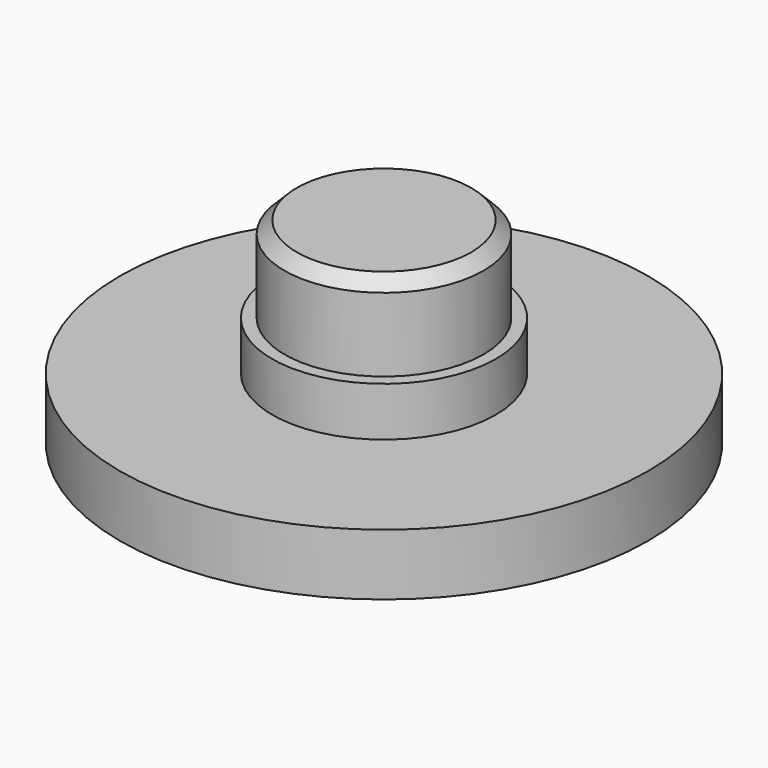
from build123d import *

# Parameters (mm, degrees)
F0_R     = 10.75
F0_R_2   = 10
F1_DEPTH = 2.5
F2_R     = 4.05
F3_DEPTH = 5.5
F4_SIZE  = 0.5
F5_R     = 4.55
F6_DEPTH = 2
F7_DEPTH = 0.5


# Not quite as in the source:
# - a feature names something its author has since deleted; it is built from what else it names


with BuildPart() as f1:
    # F0 (on Top) → F1 (new body)
    with BuildSketch(Plane.XY):
        Circle(F0_R)
        Circle(F0_R_2, mode=Mode.SUBTRACT)
        Circle(F0_R_2)
        Polygon((-0.8144098687, 5.5770273648), (3.432810713, 8.7260752933), (2.0940857055, 4.3571935282), (5.0940976108, -0.8390625077), (5.23705231, -2.0832140472), (5.8405975225, -7.3359389308), (2.7263974316, -3.992128183), (-3.2736025686, -3.992128183), (-4.4226424415, -3.4938133181), (-9.2734082358, -1.3901363628), (-4.8204831373, -0.3650653455), (-1.8204831373, 4.8310870772), align=None, mode=Mode.SUBTRACT)
        Polygon((2.0940857055, 4.3571935282), (3.432810713, 8.7260752933), (-0.8144098687, 5.5770273648), (-1.8204831373, 4.8310870772), (-4.8204831373, -0.3650653455), (-9.2734082358, -1.3901363628), (-4.4226424415, -3.4938133181), (-3.2736025686, -3.992128183), (2.7263974316, -3.992128183), (5.8405975225, -7.3359389308), (5.23705231, -2.0832140472), (5.0940976108, -0.8390625077), align=None)
    extrude(amount=F1_DEPTH)

    # F2 (on face) → F3 (join)
    with BuildSketch(Plane.XY.offset(2.5)):
        Circle(F2_R)
    extrude(amount=F3_DEPTH)

    # F4
    f4_edges = [f1.edges().sort_by_distance(p)[0] for p in [
        (-4.05, 0, 8),
    ]]
    chamfer(f4_edges, length=F4_SIZE)

    # F5 (on face) → F6 (join)
    with BuildSketch(Plane.XY.offset(2.5)):
        Circle(F5_R)
    extrude(amount=F6_DEPTH)

    # F0 (on Top) → F7 (cut)
    with BuildSketch(Plane.XY):
        Polygon((2.0940857055, 4.3571935282), (3.432810713, 8.7260752933), (-0.8144098687, 5.5770273648), (-1.8204831373, 4.8310870772), (-4.8204831373, -0.3650653455), (-9.2734082358, -1.3901363628), (-4.4226424415, -3.4938133181), (-3.2736025686, -3.992128183), (2.7263974316, -3.992128183), (5.8405975225, -7.3359389308), (5.23705231, -2.0832140472), (5.0940976108, -0.8390625077), align=None)
    extrude(amount=F7_DEPTH, mode=Mode.SUBTRACT)


solid = f1.part
